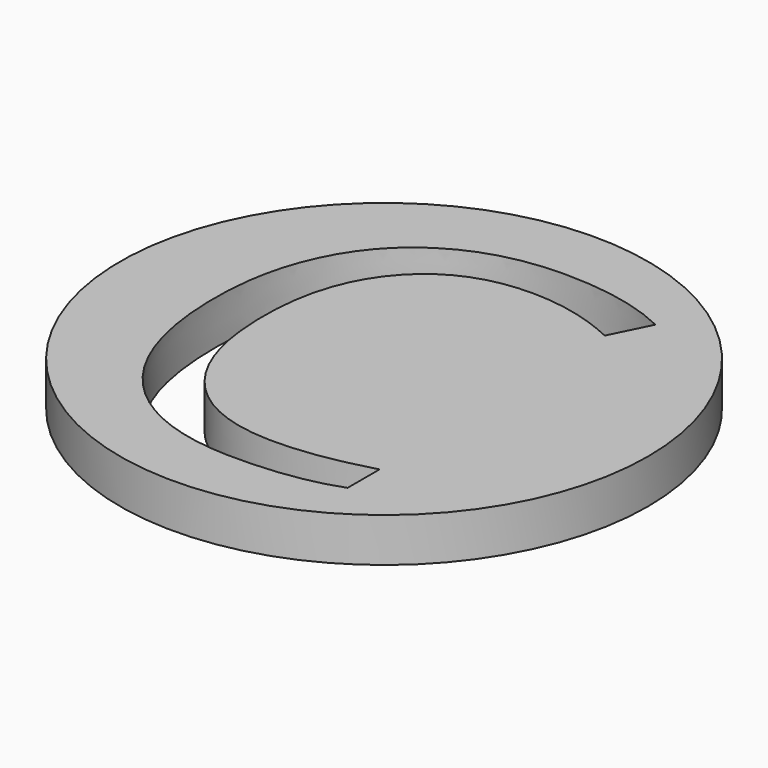
from build123d import *

# Parameters (mm, degrees)
F0_R         = 12
F1_DEPTH     = 2
F2_TEXT_SIZE = 25
F3_DEPTH     = 25


# Not quite as in the source:
# - Text() gives the source's letters only with a copy of the font that has no kerning and outlines rounded to 1/6400 em; it was checked with that copy


with BuildPart() as f1:
    # F0 (on Top) → F1 (new body)
    with BuildSketch(Plane.XY):
        Circle(F0_R)
    extrude(amount=F1_DEPTH)

    # F2 (on face) → F3 (cut)
    with BuildSketch(Plane.XY.offset(2)):
        with Locations((-9.1541550569, -9)):
            Text('C', F2_TEXT_SIZE, font='Open Sans', text_align=(TextAlign.LEFT, TextAlign.BOTTOM))
    extrude(amount=-F3_DEPTH, mode=Mode.SUBTRACT)


solid = f1.part
